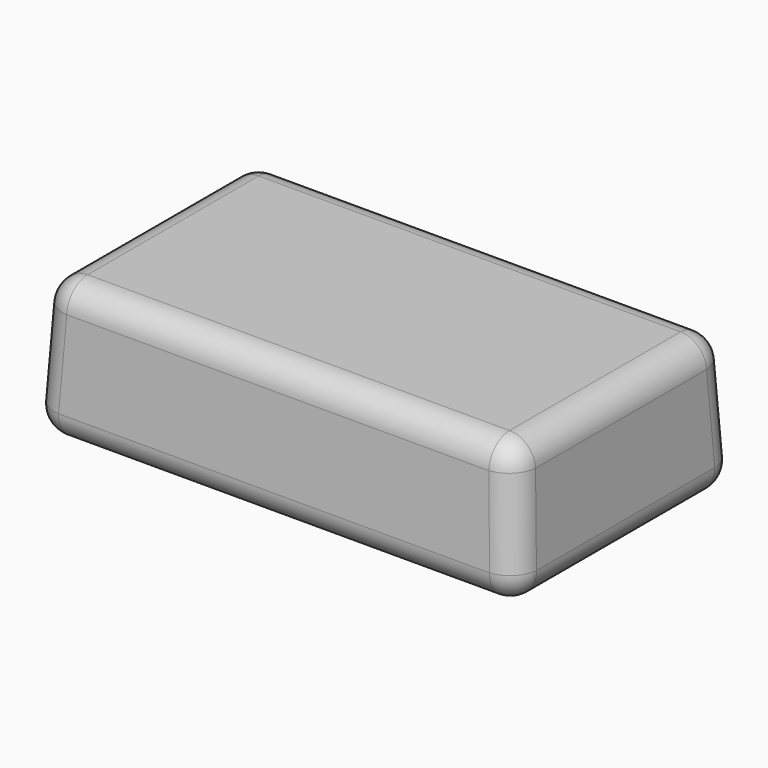
from build123d import *

# Parameters (mm, degrees)
F0_W     = 177.8
F0_H     = 101.6
F1_DEPTH = 50.8
F1_TAPER = 3
F2_R     = 9.525
F3_T     = -1.27


# Not quite as in the source:
# - a shell that OpenCascade refuses in one call is made with other operations: the cavity is built on its own and cut out


with BuildPart() as f1:
    # F0 (on Top) → F1 (new body)
    with BuildSketch(Plane.XY):
        Rectangle(F0_W, F0_H)
    extrude(amount=F1_DEPTH, taper=F1_TAPER)

    # F2
    f2_edges = [f1.edges().sort_by_distance(p)[0] for p in [
        (0, -50.8, 0),
        (87.568842, -49.468842, 25.4),
        (-87.568842, -49.468842, 25.4),
        (0, -48.137685, 50.8),
        (0, 48.137685, 50.8),
        (-86.237685, 0, 50.8),
        (86.237685, 0, 50.8),
        (88.9, 0, 0),
        (87.568842, 49.468842, 25.4),
        (0, 50.8, 0),
        (-87.568842, 49.468842, 25.4),
        (-88.9, 0, 0),
    ]]
    fillet(f2_edges, radius=F2_R)

    # F3: a shell. OpenCascade refuses it in one call, so the cavity is built on its own and cut out:
    # the body offset inwards by the wall thickness, plus a prism from it out through each open face.
    f3_core = offset(f1.part, amount=F3_T, mode=Mode.PRIVATE)
    f3_exits = [f3_core.faces().sort_by_distance(p)[0] for p in [
        (0, 0, 1.27),
    ]]
    add(f3_core, mode=Mode.SUBTRACT)
    extrude(f3_exits, amount=-F3_T, mode=Mode.SUBTRACT)


solid = f1.part
